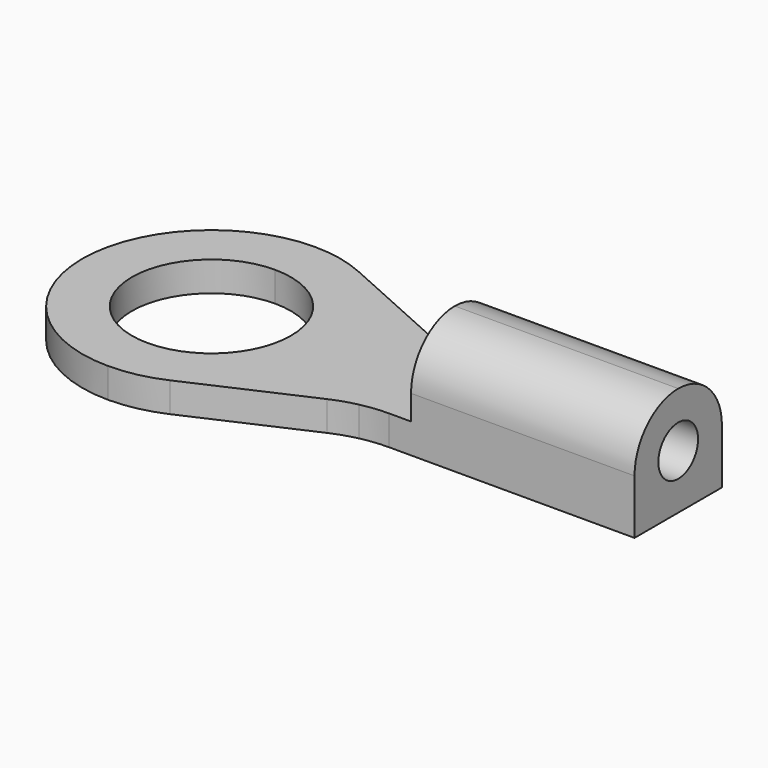
from build123d import *

# Parameters (mm, degrees)
F0_W     = 4.5
F0_H     = 2.2
F1_DEPTH = 0.6
F2_W     = 4.5
F2_H     = 2.2
F3_DEPTH = 1.6
F4_R     = 1.09999
F5_R     = 0.5
F6_DEPTH = 25


# Not quite as in the source:
# - a fillet or chamfer is up to 0.001 mm smaller than in the source, because OpenCascade refuses the exact size


with BuildPart() as f1:
    # F0 (on Top) → F1 (new body)
    with BuildSketch(Plane.XY):
        with Locations((9.75, 2.6)):
            Rectangle(F0_W, F0_H)
        with BuildLine():
            Line((7.0565025569, 1.5), (7.5, 1.5))
            Line((7.5, 1.5), (7.5, 3.7))
            Line((7.5, 3.7), (7.0565025569, 3.7))
            ThreePointArc((7.0565025569, 3.7), (6.7766250144, 3.7151076306), (6.5, 3.7602549529))
            ThreePointArc((6.5, 3.7602549529), (6.2418088438, 3.8309365837), (5.9922537502, 3.9277912239))
            Line((5.9922537502, 3.9277912239), (3.6642488067, 4.9722087761))
            ThreePointArc((3.6642488067, 4.9722087761), (4.7825497586, 4.012967286), (5.2, 2.6))
            ThreePointArc((5.2, 2.6), (4.7825497586, 1.187032714), (3.6642488067, 0.2277912239))
            Line((3.6642488067, 0.2277912239), (5.9922537502, 1.2722087761))
            ThreePointArc((5.9922537502, 1.2722087761), (6.2418088438, 1.3690634163), (6.5, 1.4397450471))
            ThreePointArc((6.5, 1.4397450471), (6.7766250144, 1.4848923694), (7.0565025569, 1.5))
        make_face()
        with BuildLine():
            ThreePointArc((2.6, 0), (3.1441769851, 0.0575855159), (3.6642488067, 0.2277912239))
            ThreePointArc((3.6642488067, 0.2277912239), (4.7825497586, 1.187032714), (5.2, 2.6))
            ThreePointArc((5.2, 2.6), (4.7825497586, 4.012967286), (3.6642488067, 4.9722087761))
            ThreePointArc((3.6642488067, 4.9722087761), (3.1441769851, 5.1424144841), (2.6, 5.2))
            Line((2.6, 5.2), (2.6, 4.2))
            ThreePointArc((2.6, 4.2), (3.7313708499, 3.7313708499), (4.2, 2.6))
            ThreePointArc((4.2, 2.6), (3.7313708499, 1.4686291501), (2.6, 1))
            Line((2.6, 1), (2.6, 0))
        make_face()
        with BuildLine():
            ThreePointArc((0, 2.6), (0.7615223689, 0.7615223689), (2.6, 0))
            Line((2.6, 0), (2.6, 1))
            ThreePointArc((2.6, 1), (1, 2.6), (2.6, 4.2))
            Line((2.6, 4.2), (2.6, 5.2))
            ThreePointArc((2.6, 5.2), (0.7615223689, 4.4384776311), (0, 2.6))
        make_face()
    extrude(amount=F1_DEPTH)

    # F2 (on face) → F3 (join)
    with BuildSketch(Plane.XY.offset(0.6)):
        with Locations((9.75, 2.6)):
            Rectangle(F2_W, F2_H)
    extrude(amount=F3_DEPTH)

    # F4 (radius 1.1 in the source; OpenCascade refuses exactly that, so slightly less here)
    f4_edges = [f1.edges().sort_by_distance(p)[0] for p in [
        (9.75, 3.7, 2.2),
        (9.75, 1.5, 2.2),
    ]]
    fillet(f4_edges, radius=F4_R)

    # F5 (on face) → F6 (cut)
    with BuildSketch(Plane.YZ.offset(12)):
        with Locations((2.6, 1.1)):
            Circle(F5_R)
    extrude(amount=-F6_DEPTH, mode=Mode.SUBTRACT)


solid = f1.part
